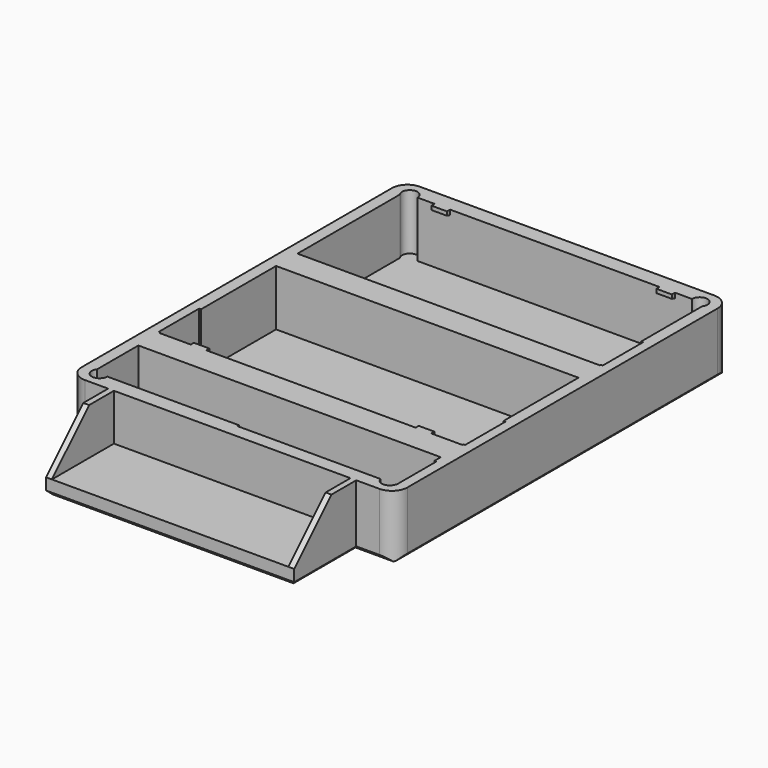
from build123d import *

# Parameters (mm, degrees)
F0_W         = 42
F0_H         = 54
F1_DEPTH     = 8
F2_W         = 39
F2_H         = 50
F3_DEPTH     = 7.2
F5_DEPTH     = 7.2
F6_W         = 20.5
F6_H         = 6.5
F6_W_2       = 18
F6_W_3       = 26.5
F7_DEPTH     = 8.001
F9_DEPTH     = 10
F10_SIZE     = 0.5
F11_T1_DEPTH = 17.5
F12_W        = 39
F12_H        = 3.45
F13_DEPTH    = 7.2
F16_DEPTH    = 1
F19_DEPTH    = 1
F20_SIZE     = 6
F22_W        = 20.5
F22_H        = 6.5
F23_DEPTH    = 0.8


# Not quite as in the source:
# - a fillet or chamfer that OpenCascade refuses, or shapes differently, is made with other operations: its cross-section is extruded or revolved along the edge and cut away or added


with BuildPart() as f1:
    # F0 (on Top) → F1 (new body)
    with BuildSketch(Plane.XY):
        with Locations((0, 27)):
            Rectangle(F0_W, F0_H)
    extrude(amount=F1_DEPTH)

    # F2 (on face) → F3 (cut)
    with BuildSketch(Plane.XY.offset(8)):
        with Locations((0, 27)):
            Rectangle(F2_W, F2_H)
    extrude(amount=-F3_DEPTH, mode=Mode.SUBTRACT)

    # F4 (on face) → F5 (cut, through all)
    with BuildSketch(Plane.XY.offset(8)):
        with BuildLine():
            Line((-19.5, 52), (-17.7, 52))
            ThreePointArc((-17.7, 52), (-19.016227766, 52.9486832981), (-19.5, 51.4))
            Line((-19.5, 51.4), (-19.5, 52))
        make_face()
        with BuildLine():
            ThreePointArc((-19.5, 51.4), (-18.383772234, 51.0513167019), (-17.7, 52))
            Line((-17.7, 52), (-19.5, 52))
            Line((-19.5, 52), (-19.5, 51.4))
        make_face()
        with BuildLine():
            Line((19.5, 52), (17.7, 52))
            ThreePointArc((17.7, 52), (18.383772234, 51.0513167019), (19.5, 51.4))
            Line((19.5, 51.4), (19.5, 52))
        make_face()
        with BuildLine():
            ThreePointArc((19.7, 52), (18.7, 53), (17.7, 52))
            Line((17.7, 52), (19.5, 52))
            Line((19.5, 52), (19.5, 51.4))
            ThreePointArc((19.5, 51.4), (19.6486832981, 51.683772234), (19.7, 52))
        make_face()
        with BuildLine():
            Line((19.5, 2), (19.5, 2.6))
            ThreePointArc((19.5, 2.6), (18.383772234, 2.9486832981), (17.7, 2))
            Line((17.7, 2), (19.5, 2))
        make_face()
        with BuildLine():
            ThreePointArc((-17.7, 2), (-18.383772234, 2.9486832981), (-19.5, 2.6))
            Line((-19.5, 2.6), (-19.5, 2))
            Line((-19.5, 2), (-17.7, 2))
        make_face()
        with BuildLine():
            Line((-19.5, 2), (-19.5, 2.6))
            ThreePointArc((-19.5, 2.6), (-19.016227766, 1.0513167019), (-17.7, 2))
            Line((-17.7, 2), (-19.5, 2))
        make_face()
        with BuildLine():
            ThreePointArc((19.7, 2), (19.6486832981, 2.316227766), (19.5, 2.6))
            Line((19.5, 2.6), (19.5, 2))
            Line((19.5, 2), (17.7, 2))
            ThreePointArc((17.7, 2), (18.7, 1), (19.7, 2))
        make_face()
    extrude(amount=-F5_DEPTH, mode=Mode.SUBTRACT)

    # F6 (on face) → F7 (cut, through all)
    with BuildSketch(Plane.XY.offset(8)):
        with Locations((9.5, 5)):
            Rectangle(F6_W, F6_H)
        with Locations((10.75, 16.1)):
            Rectangle(F6_W_2, F6_H)
        with Locations((-10.75, 16.1)):
            Rectangle(F6_W_2, F6_H)
        with Locations((6.5, 38.3)):
            Rectangle(F6_W_3, F6_H)
    extrude(amount=-F7_DEPTH, mode=Mode.SUBTRACT)

    # F8 (on face) → F9 (join)
    with BuildSketch(Plane.XZ):
        Polygon((-15.25, 2), (-15.25, 8), (-16, 8), (-16, 0), (16, 0), (16, 8), (15.25, 8), (15.25, 2), align=None)
    extrude(amount=F9_DEPTH)

    # F10
    f10_edges = [f1.edges().sort_by_distance(p)[0] for p in [
        (16, -5, 0),
        (18.5, 0, 0),
        (21, 27, 0),
        (-16, -5, 0),
        (-18.5, 0, 0),
        (-21, 27, 0),
        (0, 54, 0),
        (0, -10, 0),
    ]]
    chamfer(f10_edges, length=F10_SIZE)

    # F11: fillet of radius 2 on 4 edges, made by hand

    # F11_s2 → F11_t1 (cut)
    with BuildSketch(Plane.XY.offset(-4.5)):
        with BuildLine():
            ThreePointArc((21, 2), (20.4142135624, 0.5857864376), (19, 0))
            Line((19, 0), (21, 0))
            Line((21, 0), (21, 2))
        make_face()
        with BuildLine():
            ThreePointArc((19, 54), (20.4142135624, 53.4142135624), (21, 52))
            Line((21, 52), (21, 54))
            Line((21, 54), (19, 54))
        make_face()
        with BuildLine():
            ThreePointArc((-21, 2), (-20.4142135624, 0.5857864376), (-19, 0))
            Line((-19, 0), (-21, 0))
            Line((-21, 0), (-21, 2))
        make_face()
        with BuildLine():
            ThreePointArc((-21, 52), (-20.4142135624, 53.4142135624), (-19, 54))
            Line((-19, 54), (-21, 54))
            Line((-21, 54), (-21, 52))
        make_face()
    extrude(amount=F11_T1_DEPTH, mode=Mode.SUBTRACT)

    # F12 (on face) → F13 (join, through all)
    with BuildSketch(Plane.XY.offset(8)):
        with Locations((0, 10.975)):
            Rectangle(F12_W, F12_H)
        with Locations((0, 33.175)):
            Rectangle(F12_W, F12_H)
    extrude(amount=-F13_DEPTH)

    # F15 (on offset) → F16 (join, symmetric)
    with BuildSketch(Plane.YZ.offset(-14.5)):
        Polygon((13.2, 8), (12.7, 8), (12.7, 7.3660254038), (13.2, 7.5), align=None)
        Polygon((52, 7.3660254038), (52, 8), (51.5, 8), (51.5, 7.5), align=None)
    extrude(amount=F16_DEPTH, both=True)

    # F18 (on offset) → F19 (join, symmetric)
    with BuildSketch(Plane.YZ.offset(14.5)):
        Polygon((13.2, 7.5), (13.2, 8), (12.7, 8), (12.7, 7.3660254038), align=None)
        Polygon((51.5, 7.5), (52, 7.3660254038), (52, 8), (51.5, 8), align=None)
    extrude(amount=F19_DEPTH, both=True)

    # F20
    f20_edges = [f1.edges().sort_by_distance(p)[0] for p in [
        (-15.625, -10, 8),
        (15.625, -10, 8),
    ]]
    chamfer(f20_edges, length=F20_SIZE)

    # F22 (on face) → F23 (join)
    with BuildSketch(Plane(origin=(0, 0, 0), x_dir=(1, 0, 0), z_dir=(0, 0, -1))):
        with Locations((9.5, -5)):
            Rectangle(F22_W, F22_H)
    extrude(amount=-F23_DEPTH)


solid = f1.part
